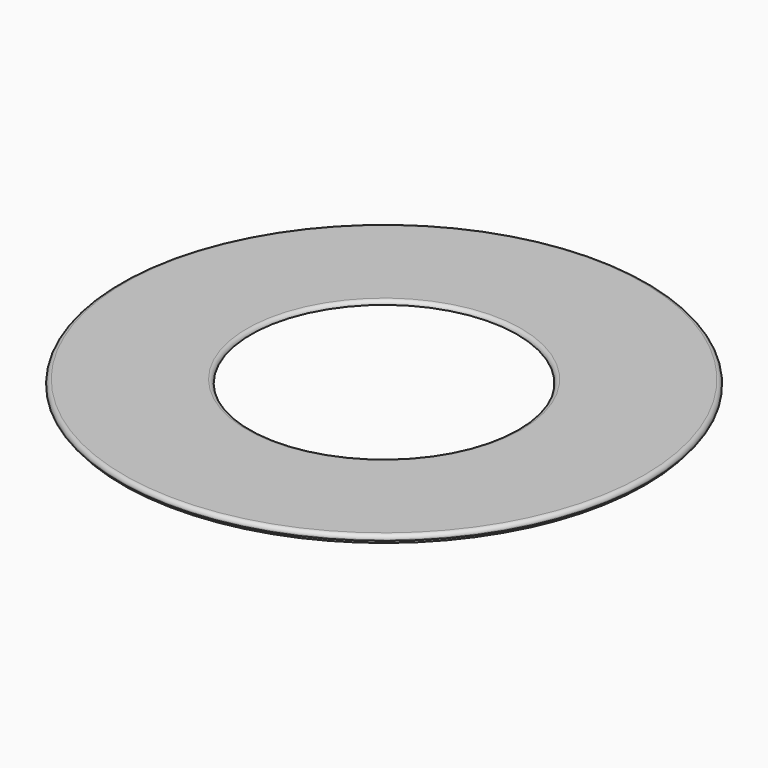
from build123d import *


# Not quite as in the source:
# - a fillet or chamfer that OpenCascade refuses, or shapes differently, is made with other operations: its cross-section is extruded or revolved along the edge and cut away or added


with BuildPart() as f1:
    # F0 (on Front) → F1 (revolve)
    with BuildSketch(Plane.XZ):
        Polygon((118, 0), (59.5, 0), (59.5, -1.75), (61.45, -1.75), (61.45, -1.65), (114.95, -1.65), (114.95, -3.75), (116.7, -3.75), (116.7, -2.25), (118, -2.25), align=None)
    revolve(axis=Axis((0, 0, -2.4080555886), (0, 0, -1)))

    # F2: fillet of radius 1.8 on 2 edges, made by hand

    # F2_s1 → F2_t2 (revolve, cut)
    with BuildSketch(Plane.XZ):
        with BuildLine():
            ThreePointArc((61.3, 0), (60.0272077939, -0.5272077939), (59.5, -1.8))
            Line((59.5, -1.8), (59.5, 0))
            Line((59.5, 0), (61.3, 0))
        make_face()
    revolve(axis=Axis((0, 0, 0), (0, 0, -1)), mode=Mode.SUBTRACT)

    # F2_s3 → F2_t4 (revolve, cut)
    with BuildSketch(Plane.XZ):
        with BuildLine():
            ThreePointArc((116.2, 0), (117.4727922061, -0.5272077939), (118, -1.8))
            Line((118, -1.8), (118, 0))
            Line((118, 0), (116.2, 0))
        make_face()
    revolve(axis=Axis((0, 0, 0), (0, 0, -1)), mode=Mode.SUBTRACT)


solid = f1.part
